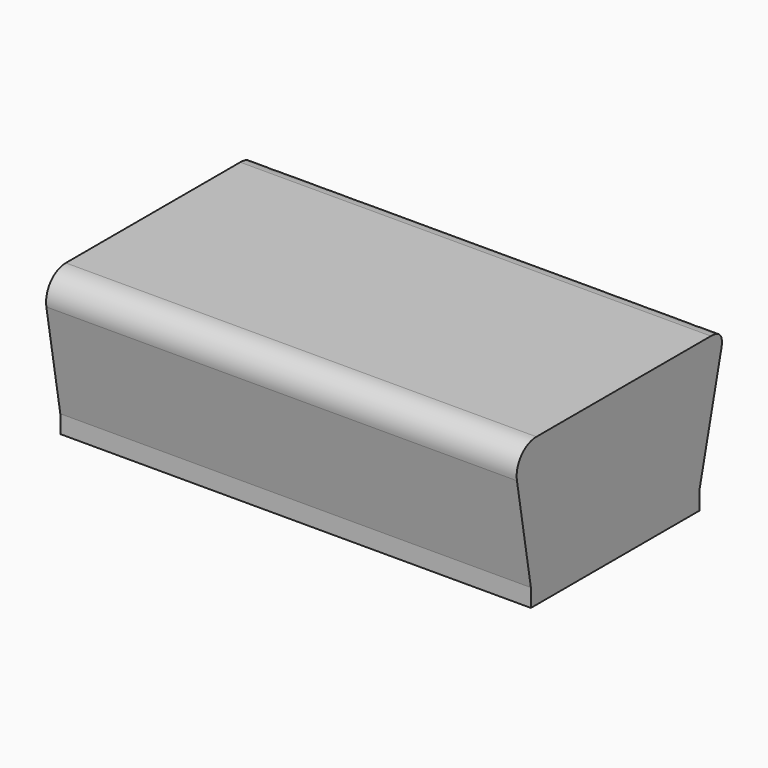
from build123d import *

# Parameters (mm, degrees)
F0_W        = 470
F0_H        = 40
F1_DEPTH    = 1050
F2_R        = 55
F3_T1_DEPTH = 1240.5148333467


# Not quite as in the source:
# - a fillet or chamfer that OpenCascade refuses, or shapes differently, is made with other operations: its cross-section is extruded or revolved along the edge and cut away or added


with BuildPart() as f1:
    # F0 (on Right) → F1 (new body)
    with BuildSketch(Plane.YZ):
        Polygon((-50, 290), (0, 0), (470, 0), (540, 290), (470, 290), align=None)
        with Locations((235, -20)):
            Rectangle(F0_W, F0_H)
    extrude(amount=F1_DEPTH)

    # F2
    f2_edges = [f1.edges().sort_by_distance(p)[0] for p in [
        (525, -50, 290),
    ]]
    fillet(f2_edges, radius=F2_R)

    # F3: fillet of radius 30 on 1 edges, made by hand

    # F3_s2 → F3_t1 (cut)
    with BuildSketch(Plane.YZ.offset(-95.2574166733)):
        with BuildLine():
            add(Edge.make_bspline(
                [(501.8970333307, 290), (540, 290), (531.0594995879, 252.9607840069)],
                knots=[0, 0, 0, 1, 1, 1], degree=2, weights=[1, 1, 1]))
            Line((531.0594995879, 252.9607840069), (540, 290))
            Line((540, 290), (501.8970333307, 290))
        make_face()
    extrude(amount=F3_T1_DEPTH, mode=Mode.SUBTRACT)


solid = f1.part
